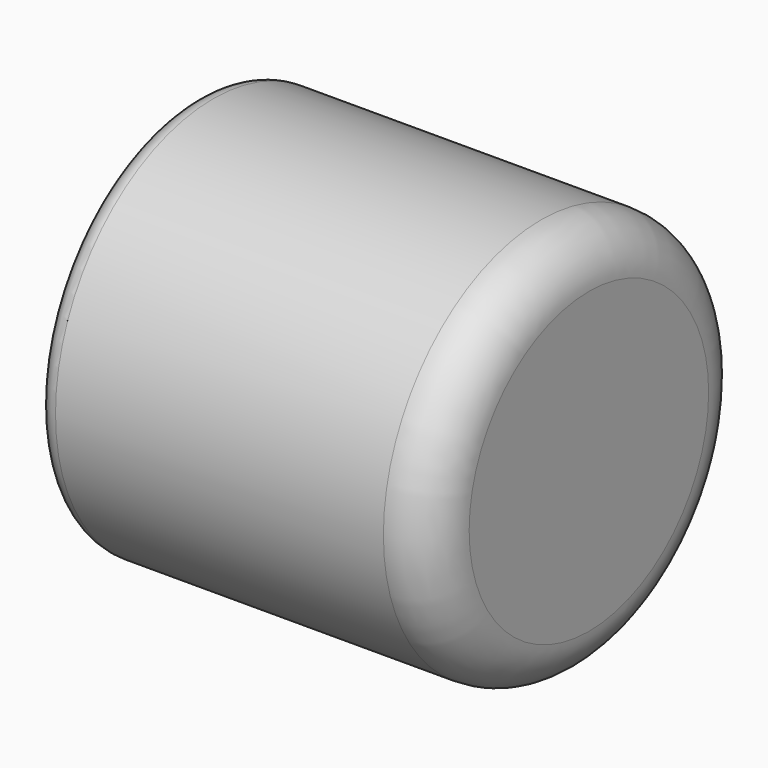
from build123d import *

# Parameters (mm, degrees)
F0_R     = 50
F1_DEPTH = 100
F2_R     = 46.2398210675
F3_DEPTH = 96
F4_R     = 12.0710678119


# Not quite as in the source:
# - a fillet or chamfer that OpenCascade refuses, or shapes differently, is made with other operations: its cross-section is extruded or revolved along the edge and cut away or added


with BuildPart() as f1:
    # F0 (on Right) → F1 (new body)
    with BuildSketch(Plane.YZ):
        Circle(F0_R)
    extrude(amount=F1_DEPTH)

    # F2 (on face) → F3 (cut)
    with BuildSketch(Plane(origin=(0, 0, 0), x_dir=(0, -1, 0), z_dir=(-1, 0, 0))):
        Circle(F2_R)
    extrude(amount=-F3_DEPTH, mode=Mode.SUBTRACT)

    # F4
    f4_edges = [f1.edges().sort_by_distance(p)[0] for p in [
        (100, -50, 0),
    ]]
    fillet(f4_edges, radius=F4_R)

    # F5: fillet of radius 5 on 1 edges, made by hand

    # F5_s1 → F5_t2 (revolve, cut)
    with BuildSketch(Plane.XY):
        with BuildLine():
            ThreePointArc((4.8438459638, 50), (1.7778310696, 48.9496269025), (0, 46.2398210675))
            Line((0, 46.2398210675), (0, 50))
            Line((0, 50), (4.8438459638, 50))
        make_face()
    revolve(axis=Axis((0, 0, 0), (1, 0, 0)), mode=Mode.SUBTRACT)


solid = f1.part
